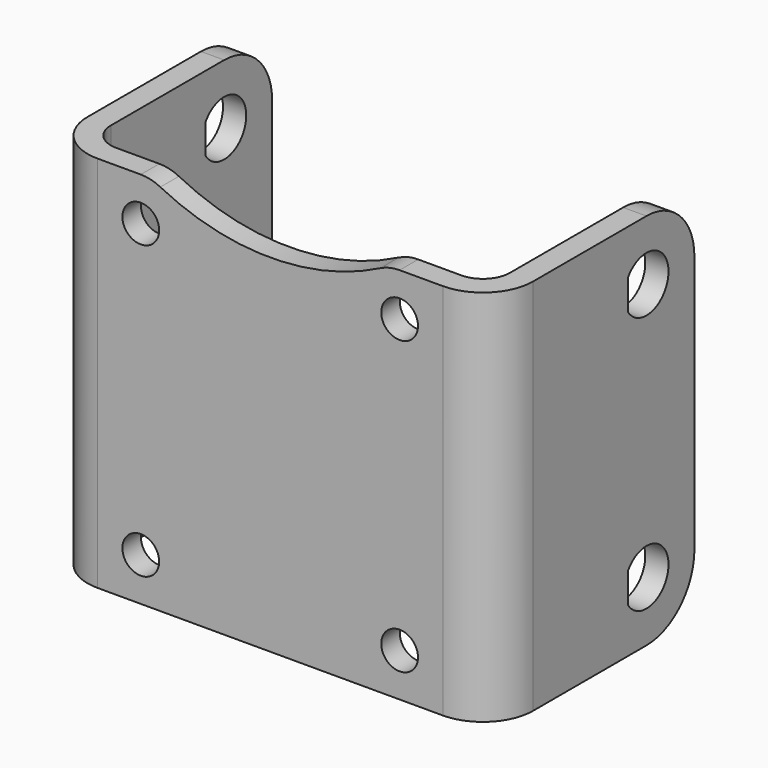
from build123d import *

# Parameters (mm, degrees)
F1_DEPTH = 27.8131016
F2_R     = 3.69316
F3_R     = 1.98374
F5_DEPTH = 32.78124
F6_R     = 1.35255
F7_DEPTH = 1.70942
F8_R     = 4.41325


with BuildPart() as f1:
    # F0 (on Top) → F1 (new body)
    with BuildSketch(Plane.XY):
        Polygon((0, 16.8191942), (0, 0), (-29.3624, 0), (-29.3624, 16.8191942), (-31.07182, 16.8191942), (-31.07182, -1.70942), (1.70942, -1.70942), (1.70942, 16.8191942), align=None)
    extrude(amount=F1_DEPTH)

    # F2
    f2_edges = [f1.edges().sort_by_distance(p)[0] for p in [
        (1.70942, -1.70942, 13.906551),
        (-31.07182, -1.70942, 13.906551),
    ]]
    fillet(f2_edges, radius=F2_R)

    # F3
    f3_edges = [f1.edges().sort_by_distance(p)[0] for p in [
        (0, 0, 13.906551),
        (-29.3624, 0, 13.906551),
    ]]
    fillet(f3_edges, radius=F3_R)

    # F4 (on face) → F5 (cut, through all)
    with BuildSketch(Plane.YZ.offset(1.70942)):
        with BuildLine():
            Line((10.7121942, 24.5224534606), (10.7121942, 22.2772497394))
            ThreePointArc((10.7121942, 22.2772497394), (14.4379442, 23.3998516), (10.7121942, 24.5224534606))
        make_face()
        with BuildLine():
            Line((10.7121942, 5.5358518606), (10.7121942, 3.2906481394))
            ThreePointArc((10.7121942, 3.2906481394), (14.4379442, 4.41325), (10.7121942, 5.5358518606))
        make_face()
    extrude(amount=-F5_DEPTH, mode=Mode.SUBTRACT)

    # F6 (on face) → F7 (cut, through all)
    with BuildSketch(Plane.XZ.offset(1.70942)):
        with BuildLine():
            ThreePointArc((-6.5960560047, 27.4691345745), (-5.8976903725, 27.7259126932), (-5.15874, 27.8131016))
            Line((-5.15874, 27.8131016), (-24.20366, 27.8131016))
            ThreePointArc((-24.20366, 27.8131016), (-23.4647096275, 27.7259126932), (-22.7663439953, 27.4691345745))
            ThreePointArc((-22.7663439953, 27.4691345745), (-14.6812, 25.5342622696), (-6.5960560047, 27.4691345745))
        make_face()
        with Locations((-24.20366, 24.6381016)):
            Circle(F6_R)
        with Locations((-5.15874, 24.6381016)):
            Circle(F6_R)
        with Locations((-24.20366, 3.175)):
            Circle(F6_R)
        with Locations((-5.15874, 3.175)):
            Circle(F6_R)
    extrude(amount=-F7_DEPTH, mode=Mode.SUBTRACT)

    # F8
    f8_edges = [f1.edges().sort_by_distance(p)[0] for p in [
        (0.85471, 16.819194, 27.813102),
        (-30.21711, 16.819194, 27.813102),
        (0.85471, 16.819194, 0),
        (-30.21711, 16.819194, 0),
    ]]
    fillet(f8_edges, radius=F8_R)


solid = f1.part
